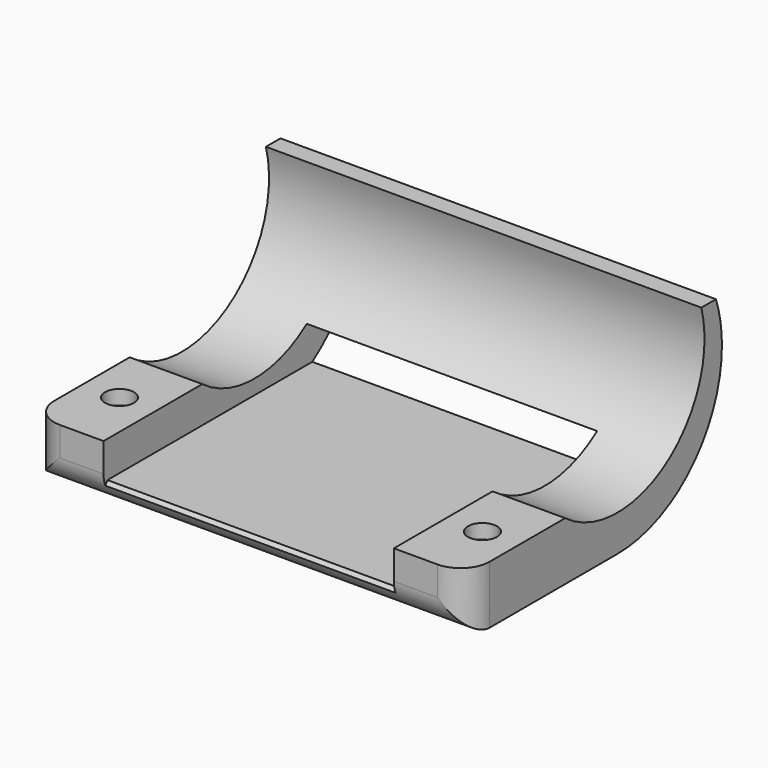
from build123d import *

# Parameters (mm, degrees)
F0_W            = 30
F0_H            = 22
F1_DEPTH        = 12
F3_DEPTH        = 30.001
F3_DEPTH_BACK   = 25
F5_START        = -25
F5_DEPTH        = 40.001
F6_R            = 2
F7_W            = 20
F7_H            = 34.384613307
F8_DEPTH        = 2.5
F9_T1_DEPTH     = 20
F11_D           = 2
F11_DEPTH       = 8
F11_CBORE_D     = 4
F11_CBORE_DEPTH = 3
F11_TIP         = 0.600860619


# Not quite as in the source:
# - a fillet or chamfer that OpenCascade refuses, or shapes differently, is made with other operations: its cross-section is extruded or revolved along the edge and cut away or added


with BuildPart() as f1:
    # F0 (on Top) → F1 (new body)
    with BuildSketch(Plane.XY):
        Rectangle(F0_W, F0_H)
    extrude(amount=F1_DEPTH)

    # F2 (on face) → F3 (cut, two sides)
    with BuildSketch(Plane(origin=(-15, 0, 0), x_dir=(0, -1, 0), z_dir=(-1, 0, 0))) as f3_sk:
        with BuildLine():
            ThreePointArc((2.5, 4), (4.7082039325, 6.6458980338), (5.5, 10))
            ThreePointArc((5.5, 10), (3.3033008589, 15.3033008589), (-2, 17.5))
            Line((-2, 17.5), (-2, 4))
            Line((-2, 4), (2.5, 4))
        make_face()
        with BuildLine():
            ThreePointArc((-2, 17.5), (3.3033008589, 15.3033008589), (5.5, 10))
            ThreePointArc((5.5, 10), (4.7082039325, 6.6458980338), (2.5, 4))
            Line((2.5, 4), (15.6530104578, 4))
            Line((15.6530104578, 4), (15.6530104578, 18.6757147312))
            Line((15.6530104578, 18.6757147312), (-2, 18.6757147312))
            Line((-2, 18.6757147312), (-2, 17.5))
        make_face()
        with BuildLine():
            Line((-2, 4), (-2, 17.5))
            ThreePointArc((-2, 17.5), (-9.1151247354, 7.6282917549), (2.5, 4))
            Line((2.5, 4), (-2, 4))
        make_face()
    extrude(amount=-F3_DEPTH, mode=Mode.SUBTRACT)
    extrude(f3_sk.sketch, amount=F3_DEPTH_BACK, mode=Mode.SUBTRACT)

    # F4 (on Right) → F5 (intersect)
    with BuildSketch(Plane.YZ.offset(F5_START)):
        with BuildLine():
            ThreePointArc((2, 0), (8.3639610307, 2.6360389693), (11, 9))
            ThreePointArc((11, 9), (8.3639610307, 15.3639610307), (2, 18))
            Line((2, 18), (2, 0))
        make_face()
        with BuildLine():
            Line((2, 0), (2, 18))
            ThreePointArc((2, 18), (-7, 9), (2, 0))
        make_face()
        with BuildLine():
            ThreePointArc((2, 0), (-7, 9), (2, 18))
            Line((2, 18), (2, 22.4318560213))
            Line((2, 22.4318560213), (-24.2340825498, 22.4318560213))
            Line((-24.2340825498, 22.4318560213), (-24.2340825498, -9.0490430593))
            Line((-24.2340825498, -9.0490430593), (2, -9.0490430593))
            Line((2, -9.0490430593), (2, 0))
        make_face()
    extrude(amount=F5_DEPTH, mode=Mode.INTERSECT)

    # F6
    f6_edges = [f1.edges().sort_by_distance(p)[0] for p in [
        (0, -11, 0),
        (-15, -11, 2),
        (15, -11, 2),
    ]]
    fillet(f6_edges, radius=F6_R)

    # F7 (on face) → F8 (cut)
    with BuildSketch(Plane.XY.offset(4)):
        with Locations((0, -1.0834368877)):
            Rectangle(F7_W, F7_H)
    extrude(amount=-F8_DEPTH, mode=Mode.SUBTRACT)

    # F9: chamfer of 0.25 on 1 edges, made by hand

    # F9_s2 → F9_t1 (cut)
    with BuildSketch(Plane.YZ.offset(-10)):
        with BuildLine():
            Line((-10.8522111232, 1.2236697613), (-10.662309407, 1.5083186711))
            Line((-10.662309407, 1.5083186711), (-10.662309407, 1.5133186711))
            ThreePointArc((-10.662309407, 1.5133186711), (-10.7994005401, 1.505), (-10.9364916731, 1.505))
            Line((-10.9364916731, 1.505), (-10.9413329023, 1.49875))
            ThreePointArc((-10.9413329023, 1.49875), (-10.9000798671, 1.3599050861), (-10.8568277766, 1.2217497324))
            Line((-10.8568277766, 1.2217497324), (-10.8522111232, 1.2236697613))
        make_face()
    extrude(amount=F9_T1_DEPTH, mode=Mode.SUBTRACT)

    # F11
    with Locations(Plane(origin=(0, 0, 0), x_dir=(1, 0, 0), z_dir=(0, 0, -1))):
        with Locations((12.5, 6.5), (-12.5, 6.5)):
            CounterBoreHole(F11_D / 2, F11_CBORE_D / 2, F11_CBORE_DEPTH, depth=F11_DEPTH)
            with Locations((0, 0, -(F11_DEPTH + F11_TIP / 2))):  # 118° drill point
                Cone(0, F11_D / 2, F11_TIP, mode=Mode.SUBTRACT)


solid = f1.part
